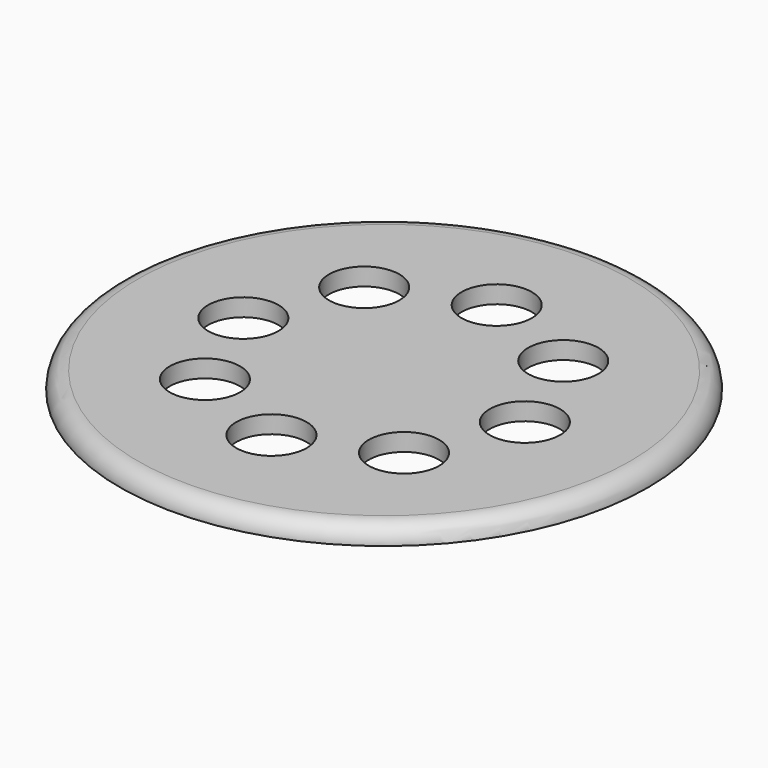
from build123d import *

# Parameters (mm, degrees)
F0_R     = 75
F2_DEPTH = 5
F3_R     = 4.99999
F1_R     = 10
F5_DEPTH = 5


# Not quite as in the source:
# - a fillet or chamfer is up to 0.001 mm smaller than in the source, because OpenCascade refuses the exact size
# - the program builds the solid bodies; features that only make, move or delete a surface that nothing else refers to are left out


with BuildPart() as f2:
    # F0 (on Top) → F2 (new body)
    with BuildSketch(Plane.XY):
        Circle(F0_R)
    extrude(amount=F2_DEPTH)

    # F3 (radius 5 in the source; OpenCascade refuses exactly that, so slightly less here)
    f3_edges = [f2.edges().sort_by_distance(p)[0] for p in [
        (-75, 0, 5),
    ]]
    fillet(f3_edges, radius=F3_R)

    # F1 (on face) → F5 (cut, through all)
    with BuildSketch(Plane.XY):
        with Locations((0, -40)):
            Circle(F1_R)
        with Locations((28.2842712475, -28.2842712475)):
            Circle(F1_R)
        with Locations((-28.2842712475, -28.2842712475)):
            Circle(F1_R)
        with Locations((-40, 0)):
            Circle(F1_R)
        with Locations((-28.2842712475, 28.2842712475)):
            Circle(F1_R)
        with Locations((0, 40)):
            Circle(F1_R)
        with Locations((28.2842712475, 28.2842712475)):
            Circle(F1_R)
        with Locations((40, 0)):
            Circle(F1_R)
    extrude(amount=F5_DEPTH, mode=Mode.SUBTRACT)


solid = f2.part
